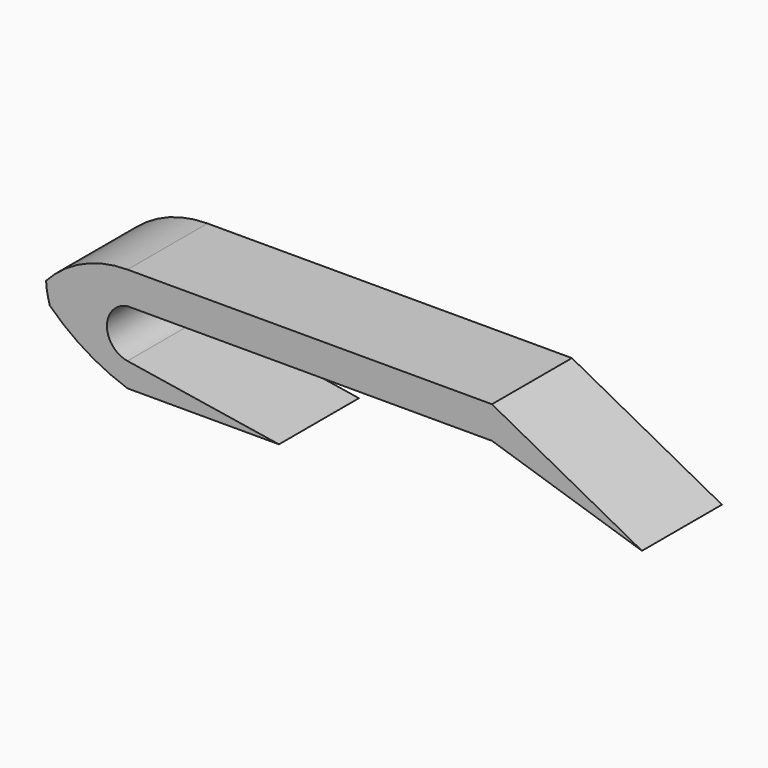
from build123d import *

# Parameters (mm, degrees)
F1_DEPTH = 25.4


# Not quite as in the source:
# - the program builds the solid bodies; features that only make, move or delete a surface that nothing else refers to are left out


with BuildPart() as f1:
    # F0 (on Front) → F1 (new body)
    with BuildSketch(Plane.XZ):
        with BuildLine():
            Line((-38.4986028075, 0), (54.1304424405, 0))
            Line((54.1304424405, 0), (92.2559946775, -12.2162923217))
            Line((92.2559946775, -12.2162923217), (54.1304424405, 8.1889424473))
            Line((54.1304424405, 8.1889424473), (-38.4986028075, 8.1889424473))
            ThreePointArc((-38.4986028075, 8.1889424473), (-49.8267048533, 5.777561047), (-59.1905941264, -1.0384666745))
            ThreePointArc((-59.1905941264, -1.0384666745), (-58.8832559342, -3.7017340098), (-58.2345825442, -6.3030168658))
            ThreePointArc((-58.2345825442, -6.3030168658), (-49.0469266103, -13.4580145444), (-38.4986028075, -18.3915607631))
            Line((-38.4986028075, -18.3915607631), (0, -18.3915607631))
            Line((0, -18.3915607631), (-38.4986028075, -12.2556750716))
            ThreePointArc((-38.4986028075, -12.2556750716), (-43.7271300367, -6.1278375358), (-38.4986028075, 0))
        make_face()
    extrude(amount=F1_DEPTH)


solid = f1.part
